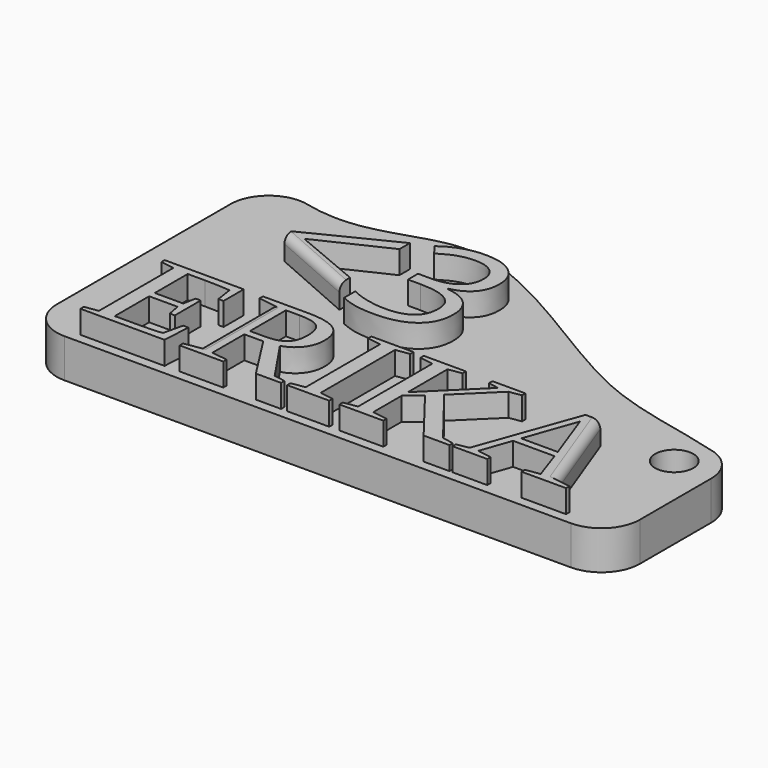
from build123d import *

# Parameters (mm, degrees)
F0_W         = 381
F0_H         = 203.2
F1_DEPTH     = 25.4
F2_TEXT_SIZE = 105.108672546
F3_DEPTH     = 15
F4_TEXT_SIZE = 118.0850590269
F5_DEPTH     = 15
F6_SCALE     = 0.2
F7_R         = 2.5
F8_DEPTH     = 25
F9_R         = 5
F10_R        = 1


# Not quite as in the source:
# - Text() gives the source's letters only with a copy of the font that has no kerning and outlines rounded to 1/6400 em; it was checked with that copy


with BuildPart() as f1:
    # F0 (on Top) → F1 (new body)
    with BuildSketch(Plane.XY):
        with Locations((190.5, 101.6)):
            Rectangle(F0_W, F0_H)
    extrude(amount=F1_DEPTH)

    # F2 (on face) → F3 (join)
    with BuildSketch(Plane.XY.offset(25.4)):
        with Locations((27.437467128, 6.274163723)):
            Text('ERIKA', F2_TEXT_SIZE, font='Tinos', text_align=(TextAlign.LEFT, TextAlign.BOTTOM))
    extrude(amount=F3_DEPTH)

    # F4 (on face) → F5 (join)
    with BuildSketch(Plane.XY.offset(25.4)):
        with Locations((54.999306798, 96.4340418577)):
            Text('<3', F4_TEXT_SIZE, font='Open Sans', text_align=(TextAlign.LEFT, TextAlign.BOTTOM))
    extrude(amount=F5_DEPTH)


with BuildPart() as f1_1:
    # F6: moved
    add(f1.part.scale(F6_SCALE))

    # F7 (on face) → F8 (cut)
    with BuildSketch(Plane(origin=(0, 0, 0), x_dir=(1, 0, 0), z_dir=(0, 0, -1))):
        with BuildLine():
            Line((76.2, -49.017958343), (76.2, -20.32))
            add(Edge.make_bspline(
                [(76.2, -20.32), (67.7625138895, -23.3060815447), (55.3182616291, -22.9760858288), (23.5792600026, -48.7792805853), (13.0098589242, -33.8729357516), (0, -40.64)],
                knots=[0, 0, 0, 0, 0.3067425209, 0.6737847669, 1, 1, 1, 1], degree=3))
            Line((0, -40.64), (76.2, -49.017958343))
        make_face()
        with Locations((70.8346217871, -17.3393078148)):
            Circle(F7_R)
    extrude(amount=-F8_DEPTH, mode=Mode.SUBTRACT)

    # F9
    f9_edges = [f1_1.edges().sort_by_distance(p)[0] for p in [
        (0, 40.64, 2.54),
        (76.2, 20.32, 2.54),
        (76.2, 0, 2.54),
        (0, 0, 2.54),
    ]]
    fillet(f9_edges, radius=F9_R)

    # F10
    f10_edges = [f1_1.edges().sort_by_distance(p)[0] for p in [
        (20.698689, 8.142735, 8.08),
        (65.374802, 8.604228, 8.08),
        (17.739935, 24.510227, 8.08),
    ]]
    fillet(f10_edges, radius=F10_R)


solid = f1_1.part
